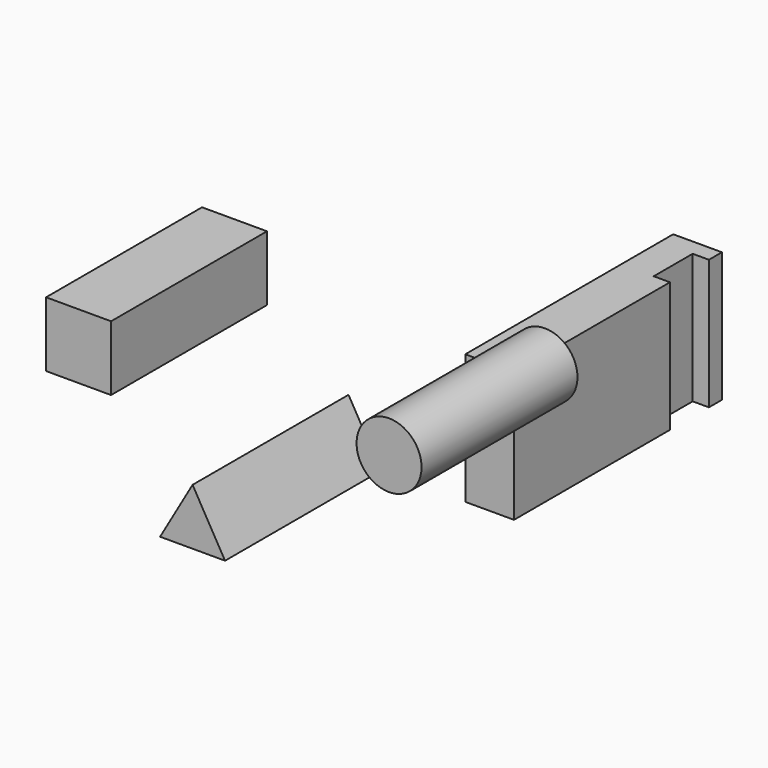
from build123d import *

# Parameters (mm, degrees)
F0_R     = 12.7
F1_DEPTH = 76.2
F0_W     = 25.4
F0_H     = 25.4
F3_DEPTH = 50.8


# Not quite as in the source:
# - a feature names something its author has since deleted; it is built from what else it names


with BuildPart() as f1:
    # F0 (on Front) → F1 (new body)
    with BuildSketch(Plane.XZ):
        with Locations((46.1565467664, 57.1670281734)):
            Circle(F0_R)
    extrude(amount=F1_DEPTH)


with BuildPart() as f1b:
    # F0 (on Front) → F1, piece 2 (new body)
    with BuildSketch(Plane.XZ):
        with Locations((-75.2221422301, 55.2151392767)):
            Rectangle(F0_W, F0_H)
    extrude(amount=F1_DEPTH)


with BuildPart() as f1c:
    # F0 (on Front) → F1, piece 3 (new body)
    with BuildSketch(Plane.XZ):
        Polygon((-43.352026199, 0), (-17.952026199, 0), (-30.652026199, 21.9970452561), align=None)
    extrude(amount=F1_DEPTH)


with BuildPart() as f3:
    # F2 (on Top) → F3 (new body)
    with BuildSketch(Plane.XY):
        Polygon((34.0507993009, 95.25), (34.0507993009, 101.6), (15.0007993009, 101.6), (15.0007993009, 0), (34.0507993009, 0), (34.0507993009, 76.2), (27.7007993009, 76.2), (27.7007993009, 95.25), align=None)
    extrude(amount=F3_DEPTH)


solid = Compound([f1.part, f1b.part, f1c.part, f3.part])
